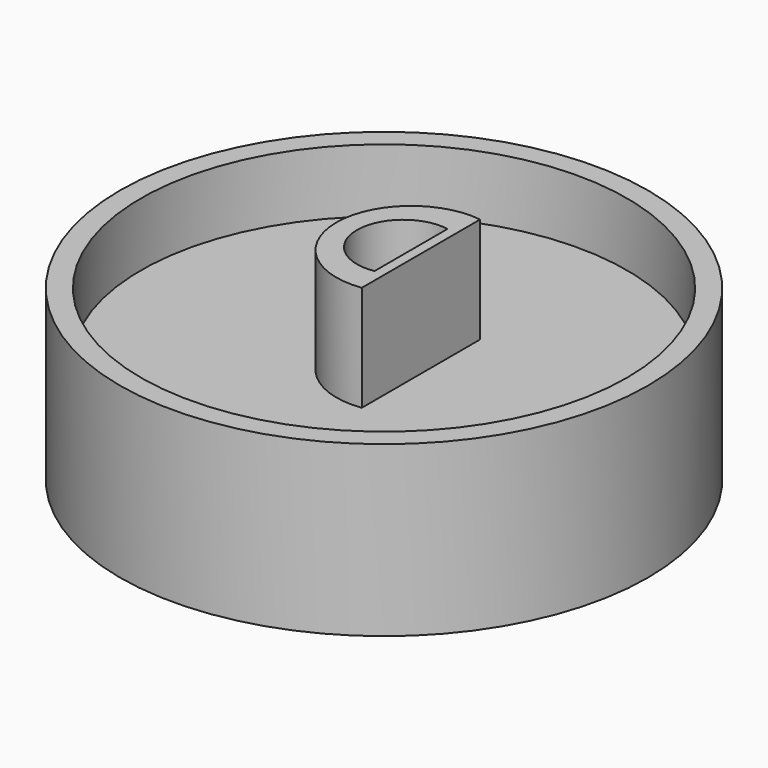
from build123d import *

# Parameters (mm, degrees)
F0_R     = 19.84375
F1_DEPTH = 6.35
F2_T     = -1.5875
F4_DEPTH = 7.9375
F6_R     = 19.84375
F7_DEPTH = 6.35


with BuildPart() as f1:
    # F0 (on Top) → F1 (new body)
    with BuildSketch(Plane.XY):
        Circle(F0_R)
    extrude(amount=F1_DEPTH)

    # F2
    f2_openings = [f1.faces().sort_by_distance(p)[0] for p in [
        (0, 0, 6.35),
    ]]
    offset(amount=F2_T, openings=f2_openings)

    # F3 (on face) → F4 (join)
    with BuildSketch(Plane.XY.offset(1.5875)):
        with BuildLine():
            Line((2.776140625, -5.55625), (2.776140625, 5.55625))
            ThreePointArc((2.776140625, 5.55625), (-3.573859375, 0), (2.776140625, -5.55625))
        make_face()
        with BuildLine():
            Line((2.032, 3.429), (2.032, -3.429))
            ThreePointArc((2.032, -3.429), (-2.032, 0), (2.032, 3.429))
        make_face(mode=Mode.SUBTRACT)
    extrude(amount=F4_DEPTH)

    # F6 (on face) → F7 (join)
    with BuildSketch(Plane(origin=(0, 0, 0), x_dir=(1, 0, 0), z_dir=(0, 0, -1))):
        Circle(F6_R)
    extrude(amount=F7_DEPTH)


solid = f1.part
